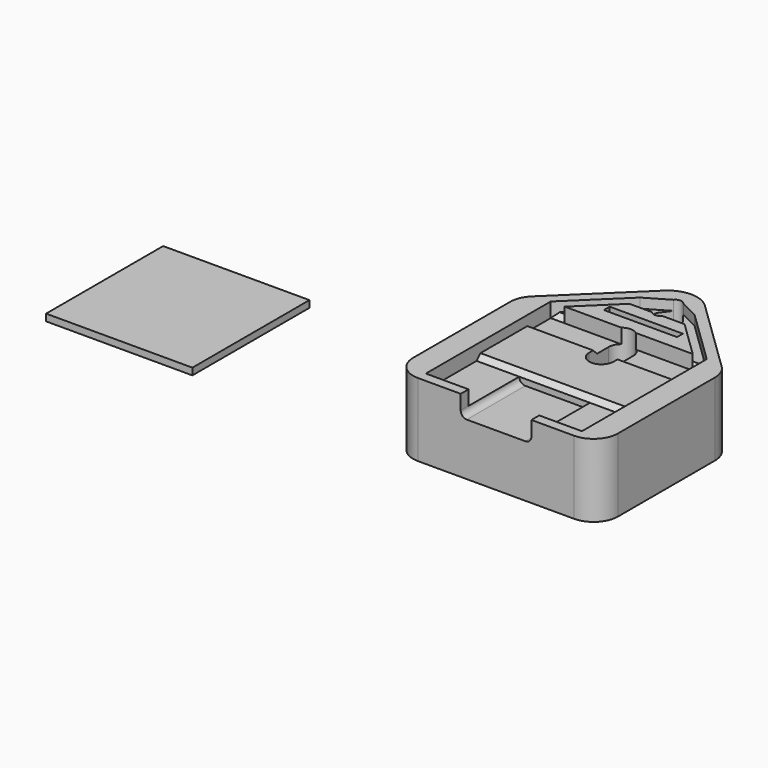
from build123d import *

# Parameters (mm, degrees)
F0_W     = 30
F0_H     = 30
F1_DEPTH = 1.4
F2_W     = 15
F2_H     = 1.5
F3_DEPTH = 15
F5_DEPTH = 2
F7_DEPTH = 15
F8_W     = 32
F8_H     = 5
F8_H_2   = 13
F9_DEPTH = 1
F10_SIZE = 0.99999


# Not quite as in the source:
# - a fillet or chamfer is up to 0.001 mm smaller than in the source, because OpenCascade refuses the exact size


with BuildPart() as f1:
    # F0 (on Top) → F1 (new body)
    with BuildSketch(Plane.XY):
        with Locations((-77.7850355953, -8.3540751795)):
            Rectangle(F0_W, F0_H)
    extrude(amount=F1_DEPTH)


with BuildPart() as f3:
    # F2 (on Top) → F3 (new body)
    with BuildSketch(Plane.XY):
        with BuildLine():
            Line((19.4800768234, 9.4733290654), (4.176092188, 24.308161329))
            ThreePointArc((4.176092188, 24.308161329), (0, 26), (-4.176092188, 24.308161329))
            Line((-4.176092188, 24.308161329), (-19.4800768234, 9.4733290654))
            ThreePointArc((-19.4800768234, 9.4733290654), (-20.6043666294, 7.8325042309), (-21, 5.8831946245))
            Line((-21, 5.8831946245), (-21, -19))
            ThreePointArc((-21, -19), (-19.5355339059, -22.5355339059), (-16, -24))
            Line((-16, -24), (16, -24))
            ThreePointArc((16, -24), (19.5355339059, -22.5355339059), (21, -19))
            Line((21, -19), (21, 5.8831946245))
            ThreePointArc((21, 5.8831946245), (20.6043666294, 7.8325042309), (19.4800768234, 9.4733290654))
        make_face()
        with BuildLine():
            ThreePointArc((-2.5, 8), (0, 10.5), (2.5, 8))
            Line((2.5, 8), (2.5, 3))
            ThreePointArc((2.5, 3), (0, 0.5), (-2.5, 3))
            Line((-2.5, 3), (-2.5, 8))
        make_face(mode=Mode.SUBTRACT)
        with Locations((0, 13.75)):
            Rectangle(F2_W, F2_H, mode=Mode.SUBTRACT)
        with BuildLine():
            ThreePointArc((-1, 22.75), (0, 23.25), (1, 22.75))
            Line((1, 22.75), (2.5, 20.75))
            ThreePointArc((2.5, 20.75), (2.75, 20), (2.5, 19.25))
            Line((2.5, 19.25), (1, 17.25))
            ThreePointArc((1, 17.25), (0, 16.75), (-1, 17.25))
            Line((-1, 17.25), (-2.5, 19.25))
            ThreePointArc((-2.5, 19.25), (-2.75, 20), (-2.5, 20.75))
            Line((-2.5, 20.75), (-1, 22.75))
        make_face(mode=Mode.SUBTRACT)
    extrude(amount=F3_DEPTH)

    # F4 (on face) → F5 (cut)
    with BuildSketch(Plane.XY.offset(15)):
        Polygon((13.1265002161, 10), (-13.1265002161, 10), (-5.6472185744, 17.25), (-1, 17.25), (-1, 22.75), (-5.6837494598, 20), (-16, 10), (-16, -22), (16, -22), (16, 10), (4.9100306693, 20.75), (1, 22.75), (1, 17.25), (5.6472185744, 17.25), align=None)
    extrude(amount=-F5_DEPTH, mode=Mode.SUBTRACT)

    # F6 (on face) → F7 (cut)
    with BuildSketch(Plane.XZ.offset(24)):
        with BuildLine():
            Line((-7.25, 15), (-7.25, 12))
            ThreePointArc((-7.25, 12), (-6.8838834765, 11.1161165235), (-6, 10.75))
            Line((-6, 10.75), (6, 10.75))
            ThreePointArc((6, 10.75), (6.8838834765, 11.1161165235), (7.25, 12))
            Line((7.25, 12), (7.25, 15))
            Line((7.25, 15), (-7.25, 15))
        make_face()
    extrude(amount=-F7_DEPTH, mode=Mode.SUBTRACT)

    # F8 (on face) → F9 (cut)
    with BuildSketch(Plane.XY.offset(13)):
        with Locations((0, 7.5)):
            Rectangle(F8_W, F8_H)
        with Locations((0, -15.5)):
            Rectangle(F8_W, F8_H_2)
    extrude(amount=-F9_DEPTH, mode=Mode.SUBTRACT)

    # F10 (size 1 in the source; OpenCascade refuses exactly that, so slightly less here)
    f10_edges = [f3.edges().sort_by_distance(p)[0] for p in [
        (-14.56325, 10, 13),
        (14.56325, 10, 13),
        (9.25, 5, 13),
        (-9.25, 5, 13),
        (0, -9, 13),
    ]]
    chamfer(f10_edges, length=F10_SIZE)


solid = Compound([f1.part, f3.part])
